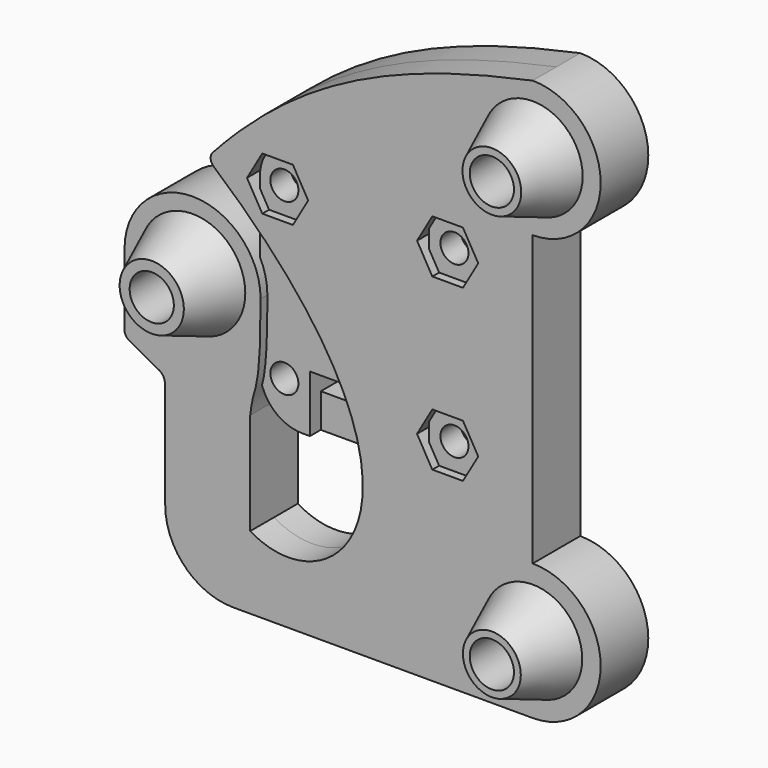
from build123d import *

# Parameters (mm, degrees)
F0_R      = 2.6
F2_DEPTH  = 3.5
F3_R      = 1.5
F4_DEPTH  = 30
F5_R      = 1
F6_R      = 2.6
F7_DEPTH  = 4
F8_R      = 1.6
F9_DEPTH  = 7.0010001
F11_DEPTH = 4
F13_R     = 6.2
F13_R_2   = 5.8806426812
F13_R_3   = 5.8298868264
F14_DEPTH = 6
F14_TAPER = 22
F15_DEPTH = 9.5010001
F1_W      = 26
F1_H      = 30
F16_DEPTH = 2.5
F17_R     = 5
F18_D     = 3.3
F19_W     = 14
F19_H     = 4
F20_DEPTH = 1.6
F19_H_2   = 2.7
F21_DEPTH = 6.0010001


# Not quite as in the source:
# - a feature names something its author has since deleted; it is built from what else it names


with BuildPart() as f2:
    # F0 (on Front) → F2 (new body, symmetric)
    with BuildSketch(Plane.XZ):
        with BuildLine():
            Line((20, -17), (20, 17))
            ThreePointArc((20, 17), (28, 25), (20, 33))
            add(Edge.make_bspline(
                [(20, 33), (3.7749062758, 29.5774657279), (-7.6347162536, 24.6316035201), (-18.301056698, 12.5704230329)],
                knots=[0, 0, 0, 0, 43.4089686498, 43.4089686498, 43.4089686498, 43.4089686498], degree=3))
            add(Edge.make_bspline(
                [(-18.301056698, 12.5704230329), (12.9501838237, -13.8033293188), (-3.0608992092, -30.5916499346), (-13.2163984158, -24.4443138838)],
                knots=[0, 0, 0, 0, 37.3623406501, 37.3623406501, 37.3623406501, 37.3623406501], degree=3))
            Line((-13.2163984158, -24.4443138838), (-13.2163984158, -12.4443138838))
            add(Edge.make_bspline(
                [(-12, 0), (-12, -10.7680466438), (-12.8143349567, -8.5643939674), (-13.2163984158, -12.4443138838)],
                knots=[0, 0, 0, 0, 12.5036224009, 12.5036224009, 12.5036224009, 12.5036224009], degree=3))
            ThreePointArc((-12, 0), (-20, 8), (-28, 0))
            Line((-28, 0), (-28, -9))
            add(Edge.make_bspline(
                [(-28, -9), (-23.8985275179, -11.5908890814), (-23.2163984158, -10.8756929968), (-23.2163984158, -13)],
                knots=[0, 0, 0, 0, 6.2356109658, 6.2356109658, 6.2356109658, 6.2356109658], degree=3))
            Line((-23.2163984158, -13), (-23.2163984158, -25))
            ThreePointArc((-23.2163984158, -25), (-20.8732526653, -30.6568542495), (-15.2163984158, -33))
            Line((-15.2163984158, -33), (20, -33))
            ThreePointArc((20, -33), (28, -25), (20, -17))
        make_face()
        with Locations((20, -25)):
            Circle(F0_R, mode=Mode.SUBTRACT)
        with Locations((-20, 0)):
            Circle(F0_R, mode=Mode.SUBTRACT)
        with Locations((20, 25)):
            Circle(F0_R, mode=Mode.SUBTRACT)
    extrude(amount=F2_DEPTH, both=True)

    # F3 (on face) → F4 (cut)
    with BuildSketch(Plane(origin=(-28, 0, 0), x_dir=(0, -1, 0), z_dir=(-1, 0, 0))):
        with Locations((0, -6.75)):
            Circle(F3_R)
    extrude(amount=-F4_DEPTH, mode=Mode.SUBTRACT)

    # F5
    f5_edges = [f2.edges().sort_by_distance(p)[0] for p in [
        (-28, 1.75, -9),
        (-28, -1.75, -9),
        (-18.301057, 1.75, 12.570423),
        (-18.301057, -1.75, 12.570423),
    ]]
    fillet(f5_edges, radius=F5_R)

    # F6 (on face) → F7 (cut)
    with BuildSketch(Plane(origin=(0, 3.5, 0), x_dir=(-1, 0, 0), z_dir=(0, 1, 0))):
        Polygon((-24.0270181276, -27.325), (-20, -29.65), (-15.9729818724, -27.325), (-15.9729818724, -22.675), (-20, -20.35), (-24.0270181276, -22.675), align=None)
        with Locations((-20, -25)):
            Circle(F6_R, mode=Mode.SUBTRACT)
        Polygon((15.9729818724, -2.325), (20, -4.65), (24.0270181276, -2.325), (24.0270181276, 2.325), (20, 4.65), (15.9729818724, 2.325), align=None)
        with Locations((20, 0)):
            Circle(F6_R, mode=Mode.SUBTRACT)
        Polygon((-24.0270181276, 22.675), (-20, 20.35), (-15.9729818724, 22.675), (-15.9729818724, 27.325), (-20, 29.65), (-24.0270181276, 27.325), align=None)
        with Locations((-20, 25)):
            Circle(F6_R, mode=Mode.SUBTRACT)
    extrude(amount=-F7_DEPTH, mode=Mode.SUBTRACT)

    # F8 (on face) → F9 (cut, through all)
    with BuildSketch(Plane.XZ.offset(3.5)):
        with Locations((10, 12)):
            Circle(F8_R)
        with Locations((-10, 12)):
            Circle(F8_R)
        with Locations((10, -8)):
            Circle(F8_R)
        with Locations((-10, -8)):
            Circle(F8_R)
    extrude(amount=-F9_DEPTH, mode=Mode.SUBTRACT)

    # F10 (on face) → F11 (cut)
    with BuildSketch(Plane.XZ.offset(3.5)):
        Polygon((-8.2, 8.8823085464), (-6.4, 12), (-8.2, 15.1176914536), (-11.8, 15.1176914536), (-13.6, 12), (-11.8, 8.8823085464), align=None)
        Polygon((13.6, 12), (11.8, 15.1176914536), (8.2, 15.1176914536), (6.4, 12), (8.2, 8.8823085464), (11.8, 8.8823085464), align=None)
        Polygon((13.6, -8), (11.8, -4.8823085464), (8.2, -4.8823085464), (6.4, -8), (8.2, -11.1176914536), (11.8, -11.1176914536), align=None)
    extrude(amount=-F11_DEPTH, mode=Mode.SUBTRACT)

    # F13 (on offset) → F14 (join)
    with BuildSketch(Plane.XZ.offset(3.5)):
        with Locations((-20, 0)):
            Circle(F13_R)
        with Locations((20, 25)):
            Circle(F13_R_2)
        with Locations((20, -25)):
            Circle(F13_R_3)
    extrude(amount=F14_DEPTH, taper=F14_TAPER)

    # F0 (on Front) → F15 (cut, through all)
    with BuildSketch(Plane.XZ):
        with Locations((20, -25)):
            Circle(F0_R)
        with Locations((20, 25)):
            Circle(F0_R)
        with Locations((-20, 0)):
            Circle(F0_R)
    extrude(amount=F15_DEPTH, mode=Mode.SUBTRACT)


with BuildPart() as f16:
    # F1 (on Front) → F16 (new body, symmetric)
    with BuildSketch(Plane.XZ):
        with Locations((0.1201688498, 2)):
            Rectangle(F1_W, F1_H)
    extrude(amount=F16_DEPTH, both=True)

    # F17
    f17_edges = [f16.edges().sort_by_distance(p)[0] for p in [
        (-12.879831, 0, 17),
        (-12.879831, 0, -13),
        (13.120169, 0, 17),
        (13.120169, 0, -13),
    ]]
    fillet(f17_edges, radius=F17_R)

    # F18 (through all)
    with Locations(Plane.XZ.offset(3.5)):
        with Locations((10, 12), (-10, 12), (-10, -8), (10, -8)):
            Hole(F18_D / 2)

    # F19 (on face) → F20 (cut)
    with BuildSketch(Plane.XZ.offset(2.5)):
        with Locations((0, 15)):
            Rectangle(F19_W, F19_H)
        with Locations((0, -11)):
            Rectangle(F19_W, F19_H)
    extrude(amount=-F20_DEPTH, mode=Mode.SUBTRACT)

    # F19 (on face) → F21 (cut, through all)
    with BuildSketch(Plane.XZ.offset(2.5)):
        with Locations((0, -7.65)):
            Rectangle(F19_W, F19_H_2)
        with Locations((0, 11.65)):
            Rectangle(F19_W, F19_H_2)
    extrude(amount=-F21_DEPTH, mode=Mode.SUBTRACT)


solid = Compound([f2.part, f16.part])
